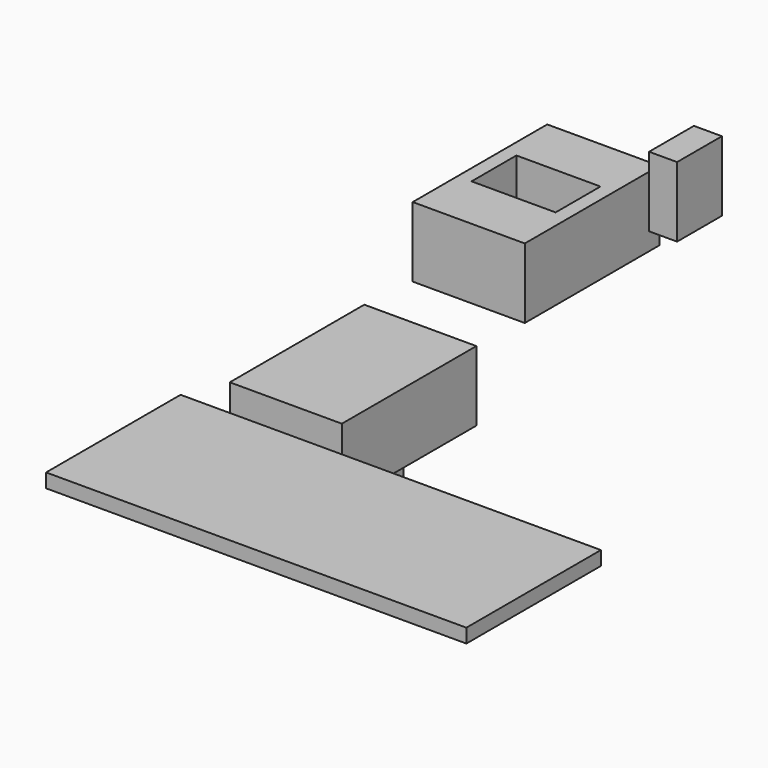
from build123d import *

# Parameters (mm, degrees)
F0_W     = 40
F0_H     = 60
F1_DEPTH = 25
F2_W     = 30
F2_H     = 20
F3_DEPTH = 25
F4_DEPTH = 25
F0_W_2   = 150
F5_DEPTH = 5
F7_W     = 20
F7_H     = 20
F8_DEPTH = 25
F2_W_2   = 10
F9_DEPTH = 25


# Not quite as in the source:
# - a feature names something its author has since deleted; it is built from what else it names


with BuildPart() as f1:
    # F0 (on Top) → F1 (new body)
    with BuildSketch(Plane.XY):
        with Locations((-29.8438598402, 49.2976413488)):
            Rectangle(F0_W, F0_H)
    extrude(amount=F1_DEPTH)

    # F2 (on face) → F3 (cut)
    with BuildSketch(Plane.XY.offset(25)):
        with Locations((-29.8438598402, 49.2976413488)):
            Rectangle(F2_W, F2_H)
    extrude(amount=-F3_DEPTH, mode=Mode.SUBTRACT)


with BuildPart() as f4:
    # F0 (on Top) → F4 (new body)
    with BuildSketch(Plane.XY):
        with Locations((-31.6961142421, -30)):
            Rectangle(F0_W, F0_H)
    extrude(amount=-F4_DEPTH)

    # F7 (on face) → F8 (join)
    with BuildSketch(Plane(origin=(0, 0, -25), x_dir=(1, 0, 0), z_dir=(0, 0, -1))):
        with Locations((-31.6961142421, 30)):
            Rectangle(F7_W, F7_H)
    extrude(amount=F8_DEPTH)


with BuildPart() as f5:
    # F0 (on Top) → F5 (new body)
    with BuildSketch(Plane.XY):
        with Locations((23.3038857579, -111.950333491)):
            Rectangle(F0_W_2, F0_H)
    extrude(amount=F5_DEPTH)


with BuildPart() as f9:
    # F2 (on face) → F9 (new body)
    with BuildSketch(Plane.XY.offset(25)):
        with Locations((17.6234441996, 56.6510467231)):
            Rectangle(F2_W_2, F2_H)
    extrude(amount=F9_DEPTH)


solid = Compound([f1.part, f4.part, f5.part, f9.part])
